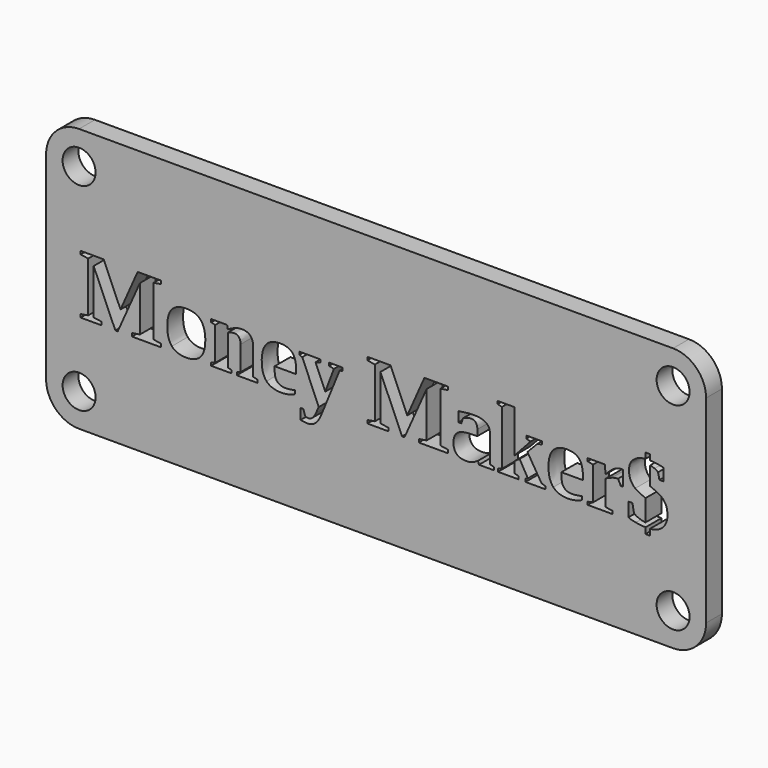
from build123d import *

# Parameters (mm, degrees)
F0_R     = 2.5
F1_DEPTH = 3


with BuildPart() as f1:
    # F0 (on Front) → F1 (new body)
    with BuildSketch(Plane.XZ):
        with BuildLine():
            ThreePointArc((0, 5), (1.4644660941, 1.4644660941), (5, 0))
            Line((5, 0), (95, 0))
            ThreePointArc((95, 0), (98.5355339059, 1.4644660941), (100, 5))
            Line((100, 5), (100, 35))
            ThreePointArc((100, 35), (98.5355339059, 38.5355339059), (95, 40))
            Line((95, 40), (5, 40))
            ThreePointArc((5, 40), (1.4644660941, 38.5355339059), (0, 35))
            Line((0, 35), (0, 5))
        make_face()
        with Locations((5, 5)):
            Circle(F0_R, mode=Mode.SUBTRACT)
        Polygon((14.2121298002, 22.434045856), (10.8580133201, 14.9074764922), (10.4924188749, 14.9074764922), (7.206319966, 22.434045856), (7.206319966, 15.5727733606), (8.4008785603, 15.3921016871), (8.4008785603, 14.9074764922), (5.2316848519, 14.9074764922), (5.2316848519, 15.3921016871), (6.3752302678, 15.5727733606), (6.3752302678, 23.15673255), (5.2316848519, 23.3310275763), (5.2316848519, 23.8156527711), (8.7324642199, 23.8156527711), (11.2767464928, 17.9555139019), (13.8741674933, 23.8156527711), (17.4472155307, 23.8156527711), (17.4472155307, 23.3310275763), (16.3057956639, 23.15673255), (16.3057956639, 15.5727733606), (17.4472155307, 15.3921016871), (17.4472155307, 14.9074764922), (13.0175712059, 14.9074764922), (13.0175712059, 15.3921016871), (14.2121298002, 15.5727733606), align=None, mode=Mode.SUBTRACT)
        with BuildLine():
            add(Edge.make_bspline(
                [(23.4295734731, 20.4912939784), (24.1235652544, 19.6644553784), (24.1235652544, 18.0617913569)],
                knots=[0, 0, 0, 1, 1, 1], degree=2))
            add(Edge.make_bspline(
                [(24.1235652544, 18.0617913569), (24.1235652544, 16.3826075678), (23.4030041094, 15.5780872333)],
                knots=[0, 0, 0, 1, 1, 1], degree=2))
            add(Edge.make_bspline(
                [(23.4030041094, 15.5780872333), (22.6824429644, 14.7735668989), (21.2009352416, 14.7735668989)],
                knots=[0, 0, 0, 1, 1, 1], degree=2))
            add(Edge.make_bspline(
                [(21.2009352416, 14.7735668989), (19.766189599, 14.7735668989), (19.0626328468, 15.5876522043)],
                knots=[0, 0, 0, 1, 1, 1], degree=2))
            add(Edge.make_bspline(
                [(19.0626328468, 15.5876522043), (18.3590760947, 16.4017375097), (18.3590760947, 18.0617913569)],
                knots=[0, 0, 0, 1, 1, 1], degree=2))
            add(Edge.make_bspline(
                [(18.3590760947, 18.0617913569), (18.3590760947, 19.7175941059), (19.0732605923, 20.5178633422)],
                knots=[0, 0, 0, 1, 1, 1], degree=2))
            add(Edge.make_bspline(
                [(19.0732605923, 20.5178633422), (19.78744509, 21.3181325784), (21.2540739691, 21.3181325784)],
                knots=[0, 0, 0, 1, 1, 1], degree=2))
            add(Edge.make_bspline(
                [(21.2540739691, 21.3181325784), (22.7355816919, 21.3181325784), (23.4295734731, 20.4912939784)],
                knots=[0, 0, 0, 1, 1, 1], degree=2))
        make_face(mode=Mode.SUBTRACT)
        with BuildLine():
            Line((27.4330452033, 21.1523397486), (27.5244438147, 20.6060736298))
            Line((27.5244438147, 20.6060736298), (27.977185773, 20.8398840308))
            add(Edge.make_bspline(
                [(27.977185773, 20.8398840308), (28.9060507298, 21.3181325784), (29.6499929148, 21.3181325784)],
                knots=[0, 0, 0, 1, 1, 1], degree=2))
            add(Edge.make_bspline(
                [(29.6499929148, 21.3181325784), (31.3780643333, 21.3181325784), (31.3780643333, 19.4774070576)],
                knots=[0, 0, 0, 1, 1, 1], degree=2))
            Line((31.3780643333, 19.4774070576), (31.3780643333, 15.5047557894))
            Line((31.3780643333, 15.5047557894), (32.0029757687, 15.3453396069))
            Line((32.0029757687, 15.3453396069), (32.0029757687, 14.9074764922))
            Line((32.0029757687, 14.9074764922), (28.8996740825, 14.9074764922))
            Line((28.8996740825, 14.9074764922), (28.8996740825, 15.3453396069))
            Line((28.8996740825, 15.3453396069), (29.4586934958, 15.5047557894))
            Line((29.4586934958, 15.5047557894), (29.4586934958, 19.2180900674))
            add(Edge.make_bspline(
                [(29.4586934958, 19.2180900674), (29.4586934958, 19.7771094807), (29.2227575457, 20.0885024239)],
                knots=[0, 0, 0, 1, 1, 1], degree=2))
            add(Edge.make_bspline(
                [(29.2227575457, 20.0885024239), (28.9868215956, 20.3998953671), (28.5489584809, 20.3998953671)],
                knots=[0, 0, 0, 1, 1, 1], degree=2))
            add(Edge.make_bspline(
                [(28.5489584809, 20.3998953671), (28.0430777951, 20.3998953671), (27.5393226584, 20.1745871625)],
                knots=[0, 0, 0, 1, 1, 1], degree=2))
            Line((27.5393226584, 20.1745871625), (27.5393226584, 15.5047557894))
            Line((27.5393226584, 15.5047557894), (28.1089698172, 15.3453396069))
            Line((28.1089698172, 15.3453396069), (28.1089698172, 14.9074764922))
            Line((28.1089698172, 14.9074764922), (25.00779368, 14.9074764922))
            Line((25.00779368, 14.9074764922), (25.00779368, 15.3453396069))
            Line((25.00779368, 15.3453396069), (25.6178262718, 15.5047557894))
            Line((25.6178262718, 15.5047557894), (25.6178262718, 20.5529349023))
            Line((25.6178262718, 20.5529349023), (25.00779368, 20.7123510848))
            Line((25.00779368, 20.7123510848), (25.00779368, 21.1523397486))
            Line((25.00779368, 21.1523397486), (27.4330452033, 21.1523397486))
        make_face(mode=Mode.SUBTRACT)
        with BuildLine():
            add(Edge.make_bspline(
                [(33.3728921638, 20.4997961748), (34.0732605923, 21.3032537347), (35.488876293, 21.3032537347)],
                knots=[0, 0, 0, 1, 1, 1], degree=2))
            add(Edge.make_bspline(
                [(35.488876293, 21.3032537347), (36.7578291059, 21.3032537347), (37.3253507156, 20.6262663463)],
                knots=[0, 0, 0, 1, 1, 1], degree=2))
            add(Edge.make_bspline(
                [(37.3253507156, 20.6262663463), (37.8928723254, 19.9492789579), (37.8928723254, 18.5209099625)],
                knots=[0, 0, 0, 1, 1, 1], degree=2))
            Line((37.8928723254, 18.5209099625), (37.8928723254, 17.9767693929))
            Line((37.8928723254, 17.9767693929), (34.617401162, 17.9767693929))
            Line((34.617401162, 17.9767693929), (34.617401162, 17.8704919379))
            add(Edge.make_bspline(
                [(34.617401162, 17.8704919379), (34.617401162, 16.8799860572), (34.7768173445, 16.4612528845)],
                knots=[0, 0, 0, 1, 1, 1], degree=2))
            add(Edge.make_bspline(
                [(34.7768173445, 16.4612528845), (34.936233527, 16.0425197117), (35.2954513249, 15.8235881544)],
                knots=[0, 0, 0, 1, 1, 1], degree=2))
            add(Edge.make_bspline(
                [(35.2954513249, 15.8235881544), (35.6546691229, 15.6046565971), (36.2795805583, 15.6046565971)],
                knots=[0, 0, 0, 1, 1, 1], degree=2))
            add(Edge.make_bspline(
                [(36.2795805583, 15.6046565971), (36.8641065609, 15.6046565971), (37.7525860847, 15.7980815652)],
                knots=[0, 0, 0, 1, 1, 1], degree=2))
            Line((37.7525860847, 15.7980815652), (37.7525860847, 15.2858242321))
            add(Edge.make_bspline(
                [(37.7525860847, 15.2858242321), (37.3891171886, 15.0668926747), (36.8077795097, 14.924480885)],
                knots=[0, 0, 0, 1, 1, 1], degree=2))
            add(Edge.make_bspline(
                [(36.8077795097, 14.924480885), (36.2264418308, 14.7820690953), (35.6737990648, 14.7820690953)],
                knots=[0, 0, 0, 1, 1, 1], degree=2))
            add(Edge.make_bspline(
                [(35.6737990648, 14.7820690953), (34.1391526144, 14.7820690953), (33.4058381749, 15.5823383315)],
                knots=[0, 0, 0, 1, 1, 1], degree=2))
            add(Edge.make_bspline(
                [(33.4058381749, 15.5823383315), (32.6725237353, 16.3826075678), (32.6725237353, 18.0617913569)],
                knots=[0, 0, 0, 1, 1, 1], degree=2))
            add(Edge.make_bspline(
                [(32.6725237353, 18.0617913569), (32.6725237353, 19.6963386149), (33.3728921638, 20.4997961748)],
                knots=[0, 0, 0, 1, 1, 1], degree=2))
        make_face(mode=Mode.SUBTRACT)
        with BuildLine():
            add(Edge.make_bspline(
                [(40.8697038402, 13.7352361635), (41.0216806008, 14.0636334995), (41.3150063766, 14.7140515241)],
                knots=[0, 0, 0, 1, 1, 1], degree=2))
            Line((41.3150063766, 14.7140515241), (38.8174861839, 20.5529349023))
            Line((38.8174861839, 20.5529349023), (38.3796230693, 20.7123510848))
            Line((38.3796230693, 20.7123510848), (38.3796230693, 21.1523397486))
            Line((38.3796230693, 21.1523397486), (41.5743233669, 21.1523397486))
            Line((41.5743233669, 21.1523397486), (41.5743233669, 20.7123510848))
            Line((41.5743233669, 20.7123510848), (40.8303811818, 20.5401816077))
            Line((40.8303811818, 20.5401816077), (42.2970100609, 17.0861643199))
            Line((42.2970100609, 17.0861643199), (43.6063483066, 20.5529349023))
            Line((43.6063483066, 20.5529349023), (42.8751594162, 20.7123510848))
            Line((42.8751594162, 20.7123510848), (42.8751594162, 21.1523397486))
            Line((42.8751594162, 21.1523397486), (44.9156865524, 21.1523397486))
            Line((44.9156865524, 21.1523397486), (44.9156865524, 20.7123510848))
            Line((44.9156865524, 20.7123510848), (44.462944594, 20.5805670406))
            Line((44.462944594, 20.5805670406), (41.9994331869, 14.5163754578))
            add(Edge.make_bspline(
                [(41.9994331869, 14.5163754578), (41.5743233669, 13.4323454167), (41.2554910018, 12.9445318982)],
                knots=[0, 0, 0, 1, 1, 1], degree=2))
            add(Edge.make_bspline(
                [(41.2554910018, 12.9445318982), (40.9366586368, 12.4567183797), (40.5476831515, 12.2144057823)],
                knots=[0, 0, 0, 1, 1, 1], degree=2))
            add(Edge.make_bspline(
                [(40.5476831515, 12.2144057823), (40.1587076661, 11.9720931849), (39.6613291767, 11.9720931849)],
                knots=[0, 0, 0, 1, 1, 1], degree=2))
            add(Edge.make_bspline(
                [(39.6613291767, 11.9720931849), (39.1235652544, 11.9720931849), (38.564545841, 12.0975005818)],
                knots=[0, 0, 0, 1, 1, 1], degree=2))
            Line((38.564545841, 12.0975005818), (38.564545841, 13.7044157015))
            Line((38.564545841, 13.7044157015), (38.9641490718, 13.7044157015))
            Line((38.9641490718, 13.7044157015), (39.2489726513, 12.8690749051))
            add(Edge.make_bspline(
                [(39.2489726513, 12.8690749051), (39.4423976194, 12.7160353699), (39.7399744934, 12.7160353699)],
                knots=[0, 0, 0, 1, 1, 1], degree=2))
            add(Edge.make_bspline(
                [(39.7399744934, 12.7160353699), (39.9929148363, 12.7160353699), (40.1852770299, 12.8350661195)],
                knots=[0, 0, 0, 1, 1, 1], degree=2))
            add(Edge.make_bspline(
                [(40.1852770299, 12.8350661195), (40.3776392235, 12.9540968692), (40.5476831515, 13.1804678483)],
                knots=[0, 0, 0, 1, 1, 1], degree=2))
            add(Edge.make_bspline(
                [(40.5476831515, 13.1804678483), (40.7177270795, 13.4068388275), (40.8697038402, 13.7352361635)],
                knots=[0, 0, 0, 1, 1, 1], degree=2))
        make_face(mode=Mode.SUBTRACT)
        with Locations((95, 5)):
            Circle(F0_R, mode=Mode.SUBTRACT)
        Polygon((57.6604789571, 22.434045856), (54.306362477, 14.9074764922), (53.9407680317, 14.9074764922), (50.6546691229, 22.434045856), (50.6546691229, 15.5727733606), (51.8492277172, 15.3921016871), (51.8492277172, 14.9074764922), (48.6800340088, 14.9074764922), (48.6800340088, 15.3921016871), (49.8235794247, 15.5727733606), (49.8235794247, 23.15673255), (48.6800340088, 23.3310275763), (48.6800340088, 23.8156527711), (52.1808133768, 23.8156527711), (54.7250956497, 17.9555139019), (57.3225166501, 23.8156527711), (60.8955646875, 23.8156527711), (60.8955646875, 23.3310275763), (59.7541448207, 23.15673255), (59.7541448207, 15.5727733606), (60.8955646875, 15.3921016871), (60.8955646875, 14.9074764922), (56.4659203628, 14.9074764922), (56.4659203628, 15.3921016871), (57.6604789571, 15.5727733606), align=None, mode=Mode.SUBTRACT)
        with BuildLine():
            add(Edge.make_bspline(
                [(63.9521042936, 21.2511777817), (64.4239761939, 21.2905004401), (64.914978036, 21.2905004401)],
                knots=[0, 0, 0, 1, 1, 1], degree=2))
            add(Edge.make_bspline(
                [(64.914978036, 21.2905004401), (67.2594586935, 21.2905004401), (67.2594586935, 19.5645545707)],
                knots=[0, 0, 0, 1, 1, 1], degree=2))
            Line((67.2594586935, 19.5645545707), (67.2594586935, 15.5047557894))
            Line((67.2594586935, 15.5047557894), (67.884370129, 15.3453396069))
            Line((67.884370129, 15.3453396069), (67.884370129, 14.9074764922))
            Line((67.884370129, 14.9074764922), (65.5866515517, 14.9074764922))
            Line((65.5866515517, 14.9074764922), (65.4399886637, 15.3857250398))
            add(Edge.make_bspline(
                [(65.4399886637, 15.3857250398), (64.9213546833, 15.0328838891), (64.5036842851, 14.903225394)],
                knots=[0, 0, 0, 1, 1, 1], degree=2))
            add(Edge.make_bspline(
                [(64.5036842851, 14.903225394), (64.0860138869, 14.7735668989), (63.6609040669, 14.7735668989)],
                knots=[0, 0, 0, 1, 1, 1], degree=2))
            add(Edge.make_bspline(
                [(63.6609040669, 14.7735668989), (61.7266543857, 14.7735668989), (61.7266543857, 16.6355479107)],
                knots=[0, 0, 0, 1, 1, 1], degree=2))
            add(Edge.make_bspline(
                [(61.7266543857, 16.6355479107), (61.7266543857, 17.3391046628), (62.0125407397, 17.7610261592)],
                knots=[0, 0, 0, 1, 1, 1], degree=2))
            add(Edge.make_bspline(
                [(62.0125407397, 17.7610261592), (62.2984270937, 18.1829476556), (62.836191016, 18.3848748201)],
                knots=[0, 0, 0, 1, 1, 1], degree=2))
            add(Edge.make_bspline(
                [(62.836191016, 18.3848748201), (63.3739549384, 18.5868019846), (64.5302536489, 18.6144341229)],
                knots=[0, 0, 0, 1, 1, 1], degree=2))
            Line((64.5302536489, 18.6144341229), (65.340087856, 18.6335640648))
            Line((65.340087856, 18.6335640648), (65.340087856, 19.5432990797))
            add(Edge.make_bspline(
                [(65.340087856, 19.5432990797), (65.340087856, 20.674091201), (64.4175995465, 20.674091201)],
                knots=[0, 0, 0, 1, 1, 1], degree=2))
            add(Edge.make_bspline(
                [(64.4175995465, 20.674091201), (63.8585801332, 20.674091201), (63.1677766756, 20.3276266977)],
                knots=[0, 0, 0, 1, 1, 1], degree=2))
            Line((63.1677766756, 20.3276266977), (62.9169618818, 19.549675727))
            Line((62.9169618818, 19.549675727), (62.4769732181, 19.549675727))
            Line((62.4769732181, 19.549675727), (62.4769732181, 21.0588155882))
            add(Edge.make_bspline(
                [(62.4769732181, 21.0588155882), (63.4802323934, 21.2118551234), (63.9521042936, 21.2511777817)],
                knots=[0, 0, 0, 1, 1, 1], degree=2))
        make_face(mode=Mode.SUBTRACT)
        Polygon((70.9876718152, 24.3470400461), (70.9876718152, 17.9023751744), (73.423551084, 20.5593115496), (72.7603797648, 20.7123510848), (72.7603797648, 21.1523397486), (75.1388692079, 21.1523397486), (75.1388692079, 20.7123510848), (74.420433612, 20.567813746), (72.9325492419, 18.9991585101), (75.0793538331, 15.5047557894), (75.6362476973, 15.3453396069), (75.6362476973, 14.9074764922), (72.6349723679, 14.9074764922), (72.6349723679, 15.3453396069), (72.998441264, 15.5047557894), (71.7507439422, 17.6898202644), (70.9876718152, 17.1584329893), (70.9876718152, 15.5047557894), (71.6040810543, 15.3453396069), (71.6040810543, 14.9074764922), (68.4752727788, 14.9074764922), (68.4752727788, 15.3453396069), (69.0661754287, 15.5047557894), (69.0661754287, 23.7476351999), (68.4285106986, 23.9070513824), (68.4285106986, 24.3470400461), align=None, mode=Mode.SUBTRACT)
        with BuildLine():
            add(Edge.make_bspline(
                [(76.8212413207, 20.4997961748), (77.5216097492, 21.3032537347), (78.9372254499, 21.3032537347)],
                knots=[0, 0, 0, 1, 1, 1], degree=2))
            add(Edge.make_bspline(
                [(78.9372254499, 21.3032537347), (80.2061782627, 21.3032537347), (80.7736998725, 20.6262663463)],
                knots=[0, 0, 0, 1, 1, 1], degree=2))
            add(Edge.make_bspline(
                [(80.7736998725, 20.6262663463), (81.3412214822, 19.9492789579), (81.3412214822, 18.5209099625)],
                knots=[0, 0, 0, 1, 1, 1], degree=2))
            Line((81.3412214822, 18.5209099625), (81.3412214822, 17.9767693929))
            Line((81.3412214822, 17.9767693929), (78.0657503188, 17.9767693929))
            Line((78.0657503188, 17.9767693929), (78.0657503188, 17.8704919379))
            add(Edge.make_bspline(
                [(78.0657503188, 17.8704919379), (78.0657503188, 16.8799860572), (78.2251665013, 16.4612528845)],
                knots=[0, 0, 0, 1, 1, 1], degree=2))
            add(Edge.make_bspline(
                [(78.2251665013, 16.4612528845), (78.3845826839, 16.0425197117), (78.7438004818, 15.8235881544)],
                knots=[0, 0, 0, 1, 1, 1], degree=2))
            add(Edge.make_bspline(
                [(78.7438004818, 15.8235881544), (79.1030182797, 15.6046565971), (79.7279297152, 15.6046565971)],
                knots=[0, 0, 0, 1, 1, 1], degree=2))
            add(Edge.make_bspline(
                [(79.7279297152, 15.6046565971), (80.3124557177, 15.6046565971), (81.2009352416, 15.7980815652)],
                knots=[0, 0, 0, 1, 1, 1], degree=2))
            Line((81.2009352416, 15.7980815652), (81.2009352416, 15.2858242321))
            add(Edge.make_bspline(
                [(81.2009352416, 15.2858242321), (80.8374663455, 15.0668926747), (80.2561286666, 14.924480885)],
                knots=[0, 0, 0, 1, 1, 1], degree=2))
            add(Edge.make_bspline(
                [(80.2561286666, 14.924480885), (79.6747909877, 14.7820690953), (79.1221482216, 14.7820690953)],
                knots=[0, 0, 0, 1, 1, 1], degree=2))
            add(Edge.make_bspline(
                [(79.1221482216, 14.7820690953), (77.5875017713, 14.7820690953), (76.8541873317, 15.5823383315)],
                knots=[0, 0, 0, 1, 1, 1], degree=2))
            add(Edge.make_bspline(
                [(76.8541873317, 15.5823383315), (76.1208728922, 16.3826075678), (76.1208728922, 18.0617913569)],
                knots=[0, 0, 0, 1, 1, 1], degree=2))
            add(Edge.make_bspline(
                [(76.1208728922, 18.0617913569), (76.1208728922, 19.6963386149), (76.8212413207, 20.4997961748)],
                knots=[0, 0, 0, 1, 1, 1], degree=2))
        make_face(mode=Mode.SUBTRACT)
        with BuildLine():
            Line((84.6825846677, 21.1523397486), (84.7569788862, 19.8557547975))
            add(Edge.make_bspline(
                [(84.7569788862, 19.8557547975), (85.473288933, 20.65283571), (86.0418733173, 21.0014257625)],
                knots=[0, 0, 0, 1, 1, 1], degree=2))
            add(Edge.make_bspline(
                [(86.0418733173, 21.0014257625), (86.6104577016, 21.3500158149), (87.0802040527, 21.3500158149)],
                knots=[0, 0, 0, 1, 1, 1], degree=2))
            Line((87.0802040527, 21.3500158149), (87.4394218506, 21.3500158149))
            Line((87.4394218506, 21.3500158149), (87.4394218506, 19.0714271795))
            Line((87.4394218506, 19.0714271795), (87.0674507581, 19.0714271795))
            Line((87.0674507581, 19.0714271795), (86.6763497237, 19.908893525))
            add(Edge.make_bspline(
                [(86.6763497237, 19.908893525), (86.2576165509, 19.908893525), (85.7262292759, 19.7260963023)],
                knots=[0, 0, 0, 1, 1, 1], degree=2))
            add(Edge.make_bspline(
                [(85.7262292759, 19.7260963023), (85.1948420009, 19.5432990797), (84.7888621227, 19.2988609332)],
                knots=[0, 0, 0, 1, 1, 1], degree=2))
            Line((84.7888621227, 19.2988609332), (84.7888621227, 15.5047557894))
            Line((84.7888621227, 15.5047557894), (85.792121298, 15.3453396069))
            Line((85.792121298, 15.3453396069), (85.792121298, 14.9074764922))
            Line((85.792121298, 14.9074764922), (82.0596570781, 14.9074764922))
            Line((82.0596570781, 14.9074764922), (82.0596570781, 15.3453396069))
            Line((82.0596570781, 15.3453396069), (82.8694912852, 15.5047557894))
            Line((82.8694912852, 15.5047557894), (82.8694912852, 20.5529349023))
            Line((82.8694912852, 20.5529349023), (82.0596570781, 20.7123510848))
            Line((82.0596570781, 20.7123510848), (82.0596570781, 21.1523397486))
            Line((82.0596570781, 21.1523397486), (84.6825846677, 21.1523397486))
        make_face(mode=Mode.SUBTRACT)
        with BuildLine():
            Line((90.8275471163, 13.8702085313), (90.8275471163, 14.7735668989))
            add(Edge.make_bspline(
                [(90.8275471163, 14.7735668989), (90.1176137169, 14.7884457426), (89.3502904917, 14.934045856)],
                knots=[0, 0, 0, 1, 1, 1], degree=2))
            add(Edge.make_bspline(
                [(89.3502904917, 14.934045856), (88.5829672665, 15.0796459693), (88.2173728213, 15.2454387992)],
                knots=[0, 0, 0, 1, 1, 1], degree=2))
            Line((88.2173728213, 15.2454387992), (88.2173728213, 17.3709878993))
            Line((88.2173728213, 17.3709878993), (88.8359076095, 17.3709878993))
            Line((88.8359076095, 17.3709878993), (89.0739691087, 16.1360438721))
            add(Edge.make_bspline(
                [(89.0739691087, 16.1360438721), (89.2737707241, 15.8639735873), (89.8349156866, 15.6514186773)],
                knots=[0, 0, 0, 1, 1, 1], degree=2))
            add(Edge.make_bspline(
                [(89.8349156866, 15.6514186773), (90.396060649, 15.4388637673), (90.8275471163, 15.4261104727)],
                knots=[0, 0, 0, 1, 1, 1], degree=2))
            Line((90.8275471163, 15.4261104727), (90.8275471163, 18.6675728505))
            add(Edge.make_bspline(
                [(90.8275471163, 18.6675728505), (89.7116338387, 19.1054359651), (89.2673940768, 19.4604026648)],
                knots=[0, 0, 0, 1, 1, 1], degree=2))
            add(Edge.make_bspline(
                [(89.2673940768, 19.4604026648), (88.8231543149, 19.8153693646), (88.5734022956, 20.334003345)],
                knots=[0, 0, 0, 1, 1, 1], degree=2))
            add(Edge.make_bspline(
                [(88.5734022956, 20.334003345), (88.3236502763, 20.8526373254), (88.3236502763, 21.6433415907)],
                knots=[0, 0, 0, 1, 1, 1], degree=2))
            add(Edge.make_bspline(
                [(88.3236502763, 21.6433415907), (88.3236502763, 22.5998386858), (89.0080770866, 23.2045574048)],
                knots=[0, 0, 0, 1, 1, 1], degree=2))
            add(Edge.make_bspline(
                [(89.0080770866, 23.2045574048), (89.6925038968, 23.8092761238), (90.8275471163, 23.9006747351)],
                knots=[0, 0, 0, 1, 1, 1], degree=2))
            Line((90.8275471163, 23.9006747351), (90.8275471163, 24.7572710225))
            Line((90.8275471163, 24.7572710225), (91.5055972793, 24.7572710225))
            Line((91.5055972793, 24.7572710225), (91.5055972793, 23.9155535788))
            add(Edge.make_bspline(
                [(91.5055972793, 23.9155535788), (92.5088564546, 23.8751681459), (93.5376222191, 23.6286044503)],
                knots=[0, 0, 0, 1, 1, 1], degree=2))
            Line((93.5376222191, 23.6286044503), (93.5376222191, 21.7751256349))
            Line((93.5376222191, 21.7751256349), (92.9339662746, 21.7751256349))
            Line((92.9339662746, 21.7751256349), (92.7214113646, 22.7252460827))
            add(Edge.make_bspline(
                [(92.7214113646, 22.7252460827), (92.5279863965, 22.9186710508), (92.1964007369, 23.0674594878)],
                knots=[0, 0, 0, 1, 1, 1], degree=2))
            add(Edge.make_bspline(
                [(92.1964007369, 23.0674594878), (91.8648150772, 23.2162479248), (91.5055972793, 23.2502567104)],
                knots=[0, 0, 0, 1, 1, 1], degree=2))
            Line((91.5055972793, 23.2502567104), (91.5055972793, 20.4934195275))
            add(Edge.make_bspline(
                [(91.5055972793, 20.4934195275), (92.3366869775, 20.1618338679), (92.6746492844, 19.9790366453)],
                knots=[0, 0, 0, 1, 1, 1], degree=2))
            add(Edge.make_bspline(
                [(92.6746492844, 19.9790366453), (93.0126115913, 19.7962394226), (93.2783052289, 19.5741195417)],
                knots=[0, 0, 0, 1, 1, 1], degree=2))
            add(Edge.make_bspline(
                [(93.2783052289, 19.5741195417), (93.5439988664, 19.3519996607), (93.7374238345, 19.0597366594)],
                knots=[0, 0, 0, 1, 1, 1], degree=2))
            add(Edge.make_bspline(
                [(93.7374238345, 19.0597366594), (93.9308488026, 18.7674736582), (94.0403145813, 18.3753098492)],
                knots=[0, 0, 0, 1, 1, 1], degree=2))
            add(Edge.make_bspline(
                [(94.0403145813, 18.3753098492), (94.1497803599, 17.9831460402), (94.1497803599, 17.4772653543)],
                knots=[0, 0, 0, 1, 1, 1], degree=2))
            add(Edge.make_bspline(
                [(94.1497803599, 17.4772653543), (94.1497803599, 16.3167155456), (93.4355958623, 15.602531048)],
                knots=[0, 0, 0, 1, 1, 1], degree=2))
            add(Edge.make_bspline(
                [(93.4355958623, 15.602531048), (92.7214113646, 14.8883465503), (91.5055972793, 14.8011990372)],
                knots=[0, 0, 0, 1, 1, 1], degree=2))
            Line((91.5055972793, 14.8011990372), (91.5055972793, 13.8702085313))
            Line((91.5055972793, 13.8702085313), (90.8275471163, 13.8702085313))
        make_face(mode=Mode.SUBTRACT)
        with Locations((5, 35)):
            Circle(F0_R, mode=Mode.SUBTRACT)
        with Locations((95, 35)):
            Circle(F0_R, mode=Mode.SUBTRACT)
    extrude(amount=F1_DEPTH)


solid = f1.part
